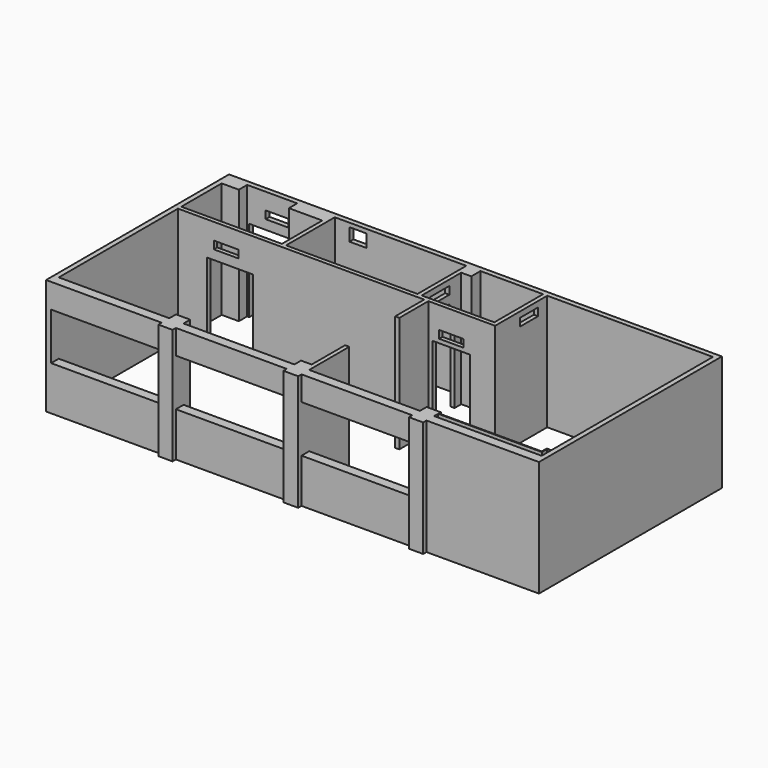
from build123d import *

# Parameters (mm, degrees)
F1_DEPTH  = 2775
F2_W      = 1100
F2_H      = 1970
F3_DEPTH  = 120
F4_W      = 100
F4_H      = 1000
F5_DEPTH  = 2775
F4_H_2    = 970
F6_W      = 5900
F6_H      = 100
F7_DEPTH  = 2775
F8_W      = 100
F8_H      = 1460
F9_DEPTH  = 2775
F10_W     = 1100
F10_H     = 1970
F11_DEPTH = 100
F12_W     = 900
F12_H     = 1970
F13_DEPTH = 100
F14_W     = 100
F14_H     = 1185
F15_DEPTH = 2775
F16_W     = 900
F16_H     = 1970
F17_DEPTH = 100
F19_DEPTH = 2775
F20_W     = 900
F20_H     = 1970
F21_DEPTH = 100
F22_W     = 2655
F22_H     = 1130
F23_DEPTH = 230
F24_W     = 2650
F24_H     = 1130
F24_W_2   = 2655
F25_DEPTH = 230
F26_W     = 406
F26_H     = 306
F27_DEPTH = 120
F28_W     = 546
F28_H     = 186
F29_DEPTH = 100
F30_W     = 586
F30_H     = 186
F31_DEPTH = 100
F32_W     = 546
F32_H     = 186
F33_DEPTH = 120
F34_W     = 586
F34_H     = 186
F35_DEPTH = 100
F37_DEPTH = 2775
F38_W     = 586
F38_H     = 186
F39_DEPTH = 100


# Not quite as in the source:
# - a feature names something its author has since deleted; it is built from what else it names


with BuildPart() as f1:
    # F0 (on Top) → F1 (new body)
    with BuildSketch(Plane.XY):
        Polygon((120, 120), (-11690, 120), (-11690, -5360), (-8920, -5360), (-8920, -5460), (-8580, -5460), (-8580, -5360), (-5925, -5360), (-5925, -5460), (-5570, -5460), (-5570, -5360), (-2915, -5360), (-2915, -5460), (-2575, -5460), (-2575, -5360), (120, -5360), align=None)
        Polygon((-5570, 0), (0, 0), (0, -5130), (-2575, -5130), (-2575, -4930), (-2915, -4930), (-2915, -5130), (-5570, -5130), (-5570, -4930), (-5925, -4930), (-5925, -5130), (-8580, -5130), (-8580, -4930), (-8920, -4930), (-8920, -5130), (-11570, -5130), (-11570, -250), (-11160, -250), (-11160, 0), (-9960, 0), (-9960, -250), (-9070, -250), (-9070, 0), (-5910, 0), (-5910, -275), (-5570, -275), align=None, mode=Mode.SUBTRACT)
    extrude(amount=F1_DEPTH)

    # F2 (on face) → F3 (cut, through all)
    with BuildSketch(Plane.XZ):
        with Locations((-10560, 985)):
            Rectangle(F2_W, F2_H)
    extrude(amount=-F3_DEPTH, mode=Mode.SUBTRACT)

    # F4 (on Top) → F5 (join, through all)
    with BuildSketch(Plane.XY):
        with Locations((-5620, -4430)):
            Rectangle(F4_W, F4_H)
    extrude(amount=F5_DEPTH)



with BuildPart() as f5:
    # F4 (on Top) → F5, piece 2 (new body, through all)
    with BuildSketch(Plane.XY):
        with Locations((-5620, -1945)):
            Rectangle(F4_W, F4_H_2)
    extrude(amount=F5_DEPTH)


with BuildPart() as f1_1:
    add(f1.part)

    add(f5.part)  # F7 merges F5
    # F6 (on Top) → F7 (join, through all)
    with BuildSketch(Plane.XY):
        with Locations((-8620, -1510)):
            Rectangle(F6_W, F6_H)
    extrude(amount=F7_DEPTH)

    # F8 (on Top) → F9 (join, through all)
    with BuildSketch(Plane.XY):
        with Locations((-9110, -730)):
            Rectangle(F8_W, F8_H)
    extrude(amount=F9_DEPTH)

    # F10 (on face) → F11 (cut, through all)
    with BuildSketch(Plane(origin=(0, -1460, 0), x_dir=(-1, 0, 0), z_dir=(0, 1, 0))):
        with Locations((10320, 985)):
            Rectangle(F10_W, F10_H)
    extrude(amount=-F11_DEPTH, mode=Mode.SUBTRACT)

    # F12 (on face) → F13 (cut, through all)
    with BuildSketch(Plane(origin=(-9160, 0, 0), x_dir=(0, -1, 0), z_dir=(-1, 0, 0))):
        with Locations((924.9999999999, 985)):
            Rectangle(F12_W, F12_H)
    extrude(amount=-F13_DEPTH, mode=Mode.SUBTRACT)

    # F14 (on Top) → F15 (join, through all)
    with BuildSketch(Plane.XY):
        with Locations((-5860, -867.5)):
            Rectangle(F14_W, F14_H)
    extrude(amount=F15_DEPTH)

    # F16 (on face) → F17 (cut, through all)
    with BuildSketch(Plane(origin=(-5910, 0, 0), x_dir=(0, -1, 0), z_dir=(-1, 0, 0))):
        with Locations((925, 985)):
            Rectangle(F16_W, F16_H)
    extrude(amount=-F17_DEPTH, mode=Mode.SUBTRACT)

    # F18 (on Top) → F19 (join, through all)
    with BuildSketch(Plane.XY):
        Polygon((-5570, -1460), (-5570, -1560), (-3970, -1560), (-3970, 0), (-4070, 0), (-4070, -1460), align=None)
    extrude(amount=F19_DEPTH)

    # F20 (on face) → F21 (cut, through all)
    with BuildSketch(Plane(origin=(0, -1460, 0), x_dir=(-1, 0, 0), z_dir=(0, 1, 0))):
        with Locations((5020, 985)):
            Rectangle(F20_W, F20_H)
    extrude(amount=-F21_DEPTH, mode=Mode.SUBTRACT)

    # F22 (on face) → F23 (cut, through all)
    with BuildSketch(Plane.XZ.offset(5360)):
        with Locations((-4242.5, 1625)):
            Rectangle(F22_W, F22_H)
    extrude(amount=-F23_DEPTH, mode=Mode.SUBTRACT)

    # F24 (on face) → F25 (cut, through all)
    with BuildSketch(Plane.XZ.offset(5360)):
        with Locations((-10245, 1625)):
            Rectangle(F24_W, F24_H)
        with Locations((-7252.5, 1625)):
            Rectangle(F24_W_2, F24_H)
    extrude(amount=-F25_DEPTH, mode=Mode.SUBTRACT)

    # F26 (on face) → F27 (cut, through all)
    with BuildSketch(Plane.XZ):
        with Locations((-8507, 2527)):
            Rectangle(F26_W, F26_H)
    extrude(amount=-F27_DEPTH, mode=Mode.SUBTRACT)

    # F28 (on face) → F29 (cut, through all)
    with BuildSketch(Plane(origin=(-4070, 0, 0), x_dir=(0, -1, 0), z_dir=(-1, 0, 0))):
        with Locations((548, 2547)):
            Rectangle(F28_W, F28_H)
    extrude(amount=-F29_DEPTH, mode=Mode.SUBTRACT)

    # F30 (on face) → F31 (cut, through all)
    with BuildSketch(Plane(origin=(-5910, 0, 0), x_dir=(0, -1, 0), z_dir=(-1, 0, 0))):
        with Locations((925, 2547)):
            Rectangle(F30_W, F30_H)
        with Locations((925, 2158)):
            Rectangle(F30_W, F30_H)
    extrude(amount=-F31_DEPTH, mode=Mode.SUBTRACT)

    # F32 (on face) → F33 (cut, through all)
    with BuildSketch(Plane.XZ):
        with Locations((-10443, 2288)):
            Rectangle(F32_W, F32_H)
    extrude(amount=-F33_DEPTH, mode=Mode.SUBTRACT)

    # F34 (on face) → F35 (cut, through all)
    with BuildSketch(Plane.XZ.offset(1560)):
        with Locations((-10417, 2288)):
            Rectangle(F34_W, F34_H)
    extrude(amount=-F35_DEPTH, mode=Mode.SUBTRACT)

    # F36 (on Top) → F37 (join, through all)
    with BuildSketch(Plane.XY):
        Polygon((-110, -4990), (-2575, -4990), (-2575, -5010), (-90, -5010), (-90, -4860), (0, -4860), (0, -4840), (-110, -4840), align=None)
    extrude(amount=F37_DEPTH)

    # F38 (on face) → F39 (cut, through all)
    with BuildSketch(Plane.XZ.offset(1560)):
        with Locations((-5020, 2158)):
            Rectangle(F38_W, F38_H)
    extrude(amount=-F39_DEPTH, mode=Mode.SUBTRACT)


solid = f1_1.part
